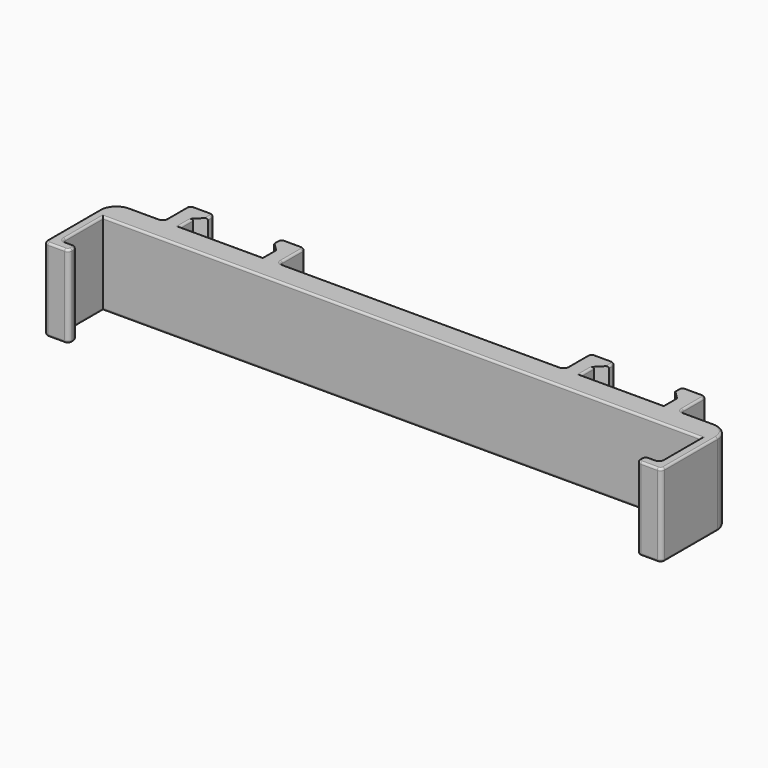
from build123d import *

# Parameters (mm, degrees)
F1_DEPTH = 5
F2_R     = 0.25


# Not quite as in the source:
# - a feature names something its author has since deleted; it is built from what else it names


with BuildPart() as f1:
    # F0 (on Top) → F1 (new body)
    with BuildSketch(Plane.XY):
        with BuildLine():
            Line((-31.75, 3), (-35.35, 3))
            ThreePointArc((-35.35, 3), (-36.7642135624, 2.4142135624), (-37.35, 1))
            Line((-37.35, 1), (-37.35, -6.95))
            ThreePointArc((-37.35, -6.95), (-37.2035533906, -7.3035533906), (-36.85, -7.45))
            Line((-36.85, -7.45), (-34.85, -7.45))
            ThreePointArc((-34.85, -7.45), (-34.4964466094, -7.3035533906), (-34.35, -6.95))
            Line((-34.35, -6.95), (-34.35, -6.7))
            ThreePointArc((-34.35, -6.7), (-34.4964466094, -6.3464466094), (-34.85, -6.2))
            Line((-34.85, -6.2), (-35.65, -6.2))
            ThreePointArc((-35.65, -6.2), (-36.0035533906, -6.0535533906), (-36.15, -5.7))
            Line((-36.15, -5.7), (-36.15, 0))
            Line((-36.15, 0), (0, 0))
            Line((0, 0), (0, 3))
            Line((0, 3), (-16.75, 3))
            ThreePointArc((-16.75, 3), (-17.1035533906, 3.1464466094), (-17.25, 3.5))
            Line((-17.25, 3.5), (-17.25, 6.5))
            ThreePointArc((-17.25, 6.5), (-17.3964466094, 6.8535533906), (-17.75, 7))
            Line((-17.75, 7), (-19.75, 7))
            ThreePointArc((-19.75, 7), (-20.1035533906, 6.8535533906), (-20.25, 6.5))
            Line((-20.25, 6.5), (-20.25, 6))
            Line((-20.25, 6), (-19.25, 5))
            Line((-19.25, 5), (-19.25, 3))
            Line((-19.25, 3), (-29.25, 3))
            Line((-29.25, 3), (-29.25, 5))
            Line((-29.25, 5), (-28.25, 6))
            Line((-28.25, 6), (-28.25, 6.5))
            ThreePointArc((-28.25, 6.5), (-28.3964466094, 6.8535533906), (-28.75, 7))
            Line((-28.75, 7), (-30.75, 7))
            ThreePointArc((-30.75, 7), (-31.1035533906, 6.8535533906), (-31.25, 6.5))
            Line((-31.25, 6.5), (-31.25, 3.5))
            ThreePointArc((-31.25, 3.5), (-31.3964466094, 3.1464466094), (-31.75, 3))
        make_face()
    extrude(amount=F1_DEPTH)

    # F2
    f2_edges = [f1.edges().sort_by_distance(p)[0] for p in [
        (-37.35, -2.975, 5),
        (-18.075, 0, 5),
        (-8.375, 3, 5),
        (-19.25, 4, 5),
        (-24.25, 3, 5),
        (-29.25, 4, 5),
    ]]
    fillet(f2_edges, radius=F2_R)

    # F3: F1 across face


with BuildPart() as f1_1:
    add(f1.part)
    add(f1.part.mirror(Plane(origin=(-20.7066751363, 1.5268952597, 0), x_dir=(1, 0, 0), z_dir=(0, 0, -1))))

    # F4: F1 across face


with BuildPart() as f1_2:
    add(f1_1.part)
    add(f1_1.part.mirror(Plane(origin=(0, 1.5, 0), x_dir=(0, 1, 0), z_dir=(1, 0, 0))))


solid = f1_2.part
